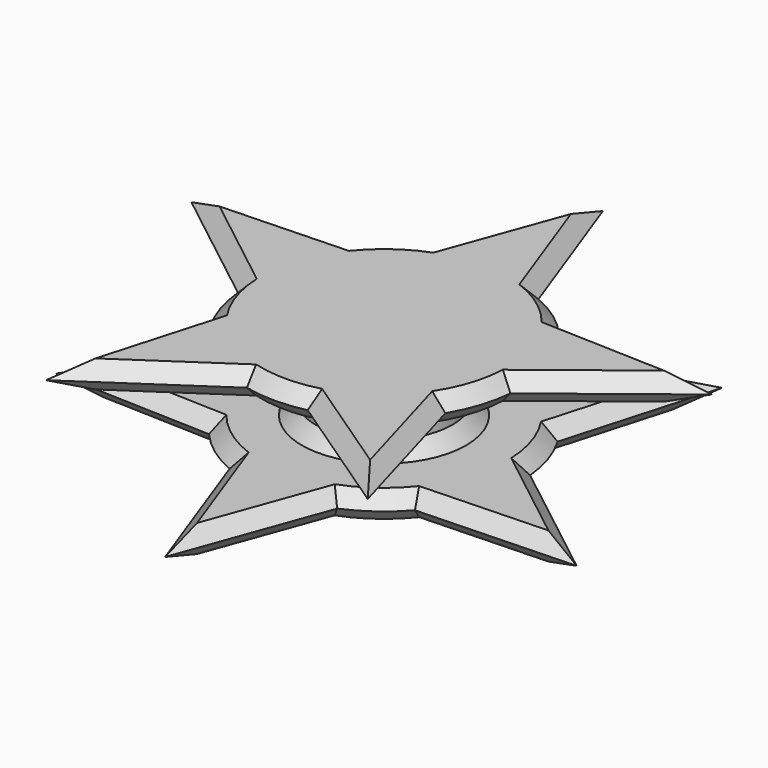
from build123d import *

# Parameters (mm, degrees)
F0_R     = 31.75
F1_DEPTH = 12.7
F5_DEPTH = 6.35
F7_DEPTH = 6.35
F8_SIZE  = 3.17499


# Not quite as in the source:
# - a fillet or chamfer is up to 0.001 mm smaller than in the source, because OpenCascade refuses the exact size


with BuildPart() as f1:
    # F0 (on Top) → F1 (new body, symmetric)
    with BuildSketch(Plane.XY):
        Circle(F0_R)
    extrude(amount=F1_DEPTH, both=True)

    # F2 (on Front) → F3 (revolve, cut)
    with BuildSketch(Plane.XZ):
        Polygon((31.75, 6.35), (15.875, 6.35), (15.875, -6.35), (31.75, -6.35), (33.2811660987, -6.35), (33.2811660987, 6.35), align=None)
    revolve(axis=Axis((0, 0, 3.175), (0, 0, 1)), mode=Mode.SUBTRACT)

    # F4 (on face) → F5 (join)
    with BuildSketch(Plane.XY.offset(12.7)):
        with BuildLine():
            ThreePointArc((0, 31.75), (6.3734153916, 31.1037309056), (12.487369908, 29.1912331494))
            Line((12.487369908, 29.1912331494), (0, 63.5))
            Line((0, 63.5), (0, 31.75))
        make_face()
        with BuildLine():
            ThreePointArc((-12.487369908, 29.1912331494), (-6.3734153916, 31.1037309056), (0, 31.75))
            Line((0, 31.75), (0, 63.5))
            Line((0, 63.5), (-12.487369908, 29.1912331494))
        make_face()
        with BuildLine():
            ThreePointArc((-31.621322022, -2.8556073925), (-30.1960443924, 9.8112895714), (-23.9037029888, 20.8967816523))
            Line((-23.9037029888, 20.8967816523), (-60.3920887847, 19.6225791428))
            Line((-60.3920887847, 19.6225791428), (-31.621322022, -2.8556073925))
        make_face()
        with BuildLine():
            Line((-37.3243635206, -51.3725791428), (-7.0556818708, -30.9560955764))
            ThreePointArc((-7.0556818708, -30.9560955764), (-18.6621817603, -25.6862895714), (-27.2606708121, -16.2763118327))
            Line((-27.2606708121, -16.2763118327), (-37.3243635206, -51.3725791428))
        make_face()
        with BuildLine():
            Line((37.3243635206, -51.3725791428), (27.2606708121, -16.2763118327))
            ThreePointArc((27.2606708121, -16.2763118327), (18.6621817603, -25.6862895714), (7.0556818708, -30.9560955764))
            Line((7.0556818708, -30.9560955764), (37.3243635206, -51.3725791428))
        make_face()
        with BuildLine():
            ThreePointArc((23.9037029888, 20.8967816523), (29.7237705372, 11.160643577), (31.75, 0))
            ThreePointArc((31.75, 0), (31.7178141917, -1.4292525671), (31.621322022, -2.8556073925))
            Line((31.621322022, -2.8556073925), (60.3920887847, 19.6225791428))
            Line((60.3920887847, 19.6225791428), (23.9037029888, 20.8967816523))
        make_face()
    extrude(amount=-F5_DEPTH)

    # F6 (on face) → F7 (join)
    with BuildSketch(Plane(origin=(0, 0, -12.7), x_dir=(1, 0, 0), z_dir=(0, 0, -1))):
        with BuildLine():
            ThreePointArc((-12.487369908, 29.1912331494), (-6.3734153916, 31.1037309056), (0, 31.75))
            Line((0, 31.75), (0, 63.5))
            Line((0, 63.5), (-12.487369908, 29.1912331494))
        make_face()
        with BuildLine():
            ThreePointArc((0, 31.75), (6.3734153916, 31.1037309056), (12.487369908, 29.1912331494))
            Line((12.487369908, 29.1912331494), (0, 63.5))
            Line((0, 63.5), (0, 31.75))
        make_face()
        with BuildLine():
            ThreePointArc((-31.621322022, -2.8556073925), (-30.1960443924, 9.8112895714), (-23.9037029888, 20.8967816523))
            Line((-23.9037029888, 20.8967816523), (-60.3920887847, 19.6225791428))
            Line((-60.3920887847, 19.6225791428), (-31.621322022, -2.8556073925))
        make_face()
        with BuildLine():
            ThreePointArc((23.9037029888, 20.8967816523), (29.7237705372, 11.160643577), (31.75, 0))
            ThreePointArc((31.75, 0), (31.7178141917, -1.4292525671), (31.621322022, -2.8556073925))
            Line((31.621322022, -2.8556073925), (60.3920887847, 19.6225791428))
            Line((60.3920887847, 19.6225791428), (23.9037029888, 20.8967816523))
        make_face()
        with BuildLine():
            Line((-37.3243635206, -51.3725791428), (-7.0556818708, -30.9560955764))
            ThreePointArc((-7.0556818708, -30.9560955764), (-18.6621817603, -25.6862895714), (-27.2606708121, -16.2763118327))
            Line((-27.2606708121, -16.2763118327), (-37.3243635206, -51.3725791428))
        make_face()
        with BuildLine():
            Line((37.3243635206, -51.3725791428), (27.2606708121, -16.2763118327))
            ThreePointArc((27.2606708121, -16.2763118327), (18.6621817603, -25.6862895714), (7.0556818708, -30.9560955764))
            Line((7.0556818708, -30.9560955764), (37.3243635206, -51.3725791428))
        make_face()
    extrude(amount=-F7_DEPTH)

    # F8 (size 3.175 in the source; OpenCascade refuses exactly that, so slightly less here)
    f8_edges = [f1.edges().sort_by_distance(p)[0] for p in [
        (18.662182, 25.68629, 12.7),
        (6.243685, 46.345617, 12.7),
        (-6.243685, 46.345617, 12.7),
        (-18.662182, 25.68629, 12.7),
        (-42.147896, 20.25968, 12.7),
        (-46.006705, 8.383486, 12.7),
        (-30.196044, -9.81129, 12.7),
        (-32.292517, -33.824445, 12.7),
        (-22.190023, -41.164337, 12.7),
        (0, -31.75, 12.7),
        (22.190023, -41.164337, 12.7),
        (32.292517, -33.824445, 12.7),
        (30.196044, -9.81129, 12.7),
        (46.006705, 8.383486, 12.7),
        (42.147896, 20.25968, 12.7),
        (30.196044, 9.81129, -6.35),
        (46.006705, -8.383486, -6.35),
        (42.147896, -20.25968, -6.35),
        (18.662182, -25.68629, -6.35),
        (6.243685, -46.345617, -6.35),
        (-6.243685, -46.345617, -6.35),
        (-18.662182, -25.68629, -6.35),
        (-42.147896, -20.25968, -6.35),
        (-46.006705, -8.383486, -6.35),
        (-30.196044, 9.81129, -6.35),
        (-32.292517, 33.824445, -6.35),
        (-22.190023, 41.164337, -6.35),
        (0, 31.75, -6.35),
        (22.190023, 41.164337, -6.35),
        (32.292517, 33.824445, -6.35),
        (-15.875, 0, -6.35),
        (18.662182, 25.68629, 6.35),
        (6.243685, 46.345617, 6.35),
        (-6.243685, 46.345617, 6.35),
        (-18.662182, 25.68629, 6.35),
        (-42.147896, 20.25968, 6.35),
        (-46.006705, 8.383486, 6.35),
        (-30.196044, -9.81129, 6.35),
        (-32.292517, -33.824445, 6.35),
        (-22.190023, -41.164337, 6.35),
        (0, -31.75, 6.35),
        (22.190023, -41.164337, 6.35),
        (32.292517, -33.824445, 6.35),
        (30.196044, -9.81129, 6.35),
        (46.006705, 8.383486, 6.35),
        (42.147896, 20.25968, 6.35),
        (-15.875, 0, 6.35),
        (30.196044, 9.81129, -12.7),
        (32.292517, 33.824445, -12.7),
        (22.190023, 41.164337, -12.7),
        (0, 31.75, -12.7),
        (-22.190023, 41.164337, -12.7),
        (-32.292517, 33.824445, -12.7),
        (-30.196044, 9.81129, -12.7),
        (-46.006705, -8.383486, -12.7),
        (-42.147896, -20.25968, -12.7),
        (-18.662182, -25.68629, -12.7),
        (-6.243685, -46.345617, -12.7),
        (6.243685, -46.345617, -12.7),
        (18.662182, -25.68629, -12.7),
        (42.147896, -20.25968, -12.7),
        (46.006705, -8.383486, -12.7),
    ]]
    chamfer(f8_edges, length=F8_SIZE)


solid = f1.part
